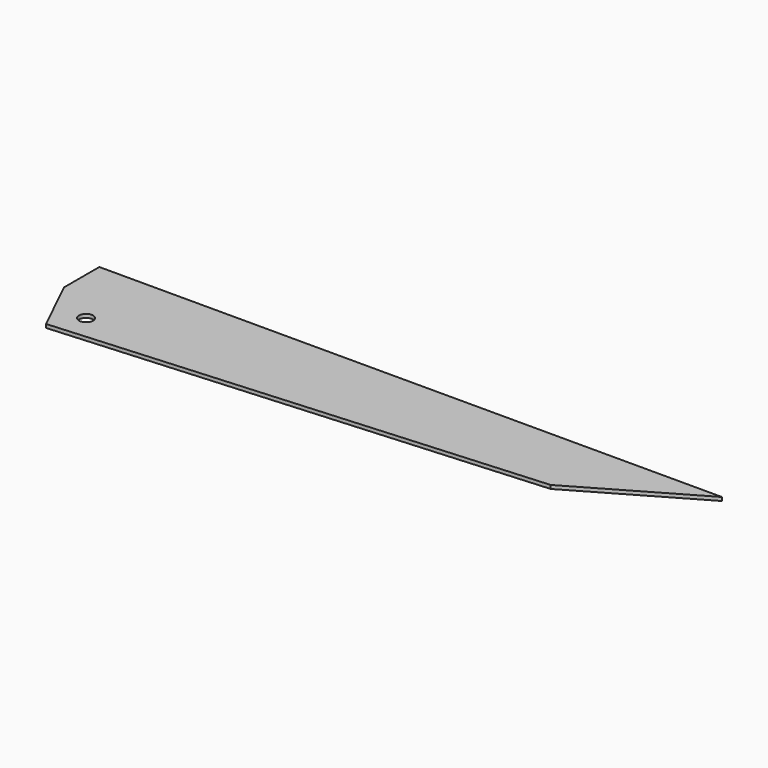
from build123d import *

# Parameters (mm, degrees)
F0_R     = 22.225
F0_R_2   = 6.35
F1_DEPTH = 3.175


# Not quite as in the source:
# - a feature names something its author has since deleted; it is built from what else it names


with BuildPart() as f1:
    # F0 (on Top) → F1 (new body)
    with BuildSketch(Plane.XY):
        Polygon((-217.8399659125, 274.6944633329), (-274.3403279131, 274.6944633329), (-249.4802269343, 223.6304721332), (-194.8479709943, 227.4676629604), align=None)
        with Locations((-233.2169740796, 248.1006040146)):
            Circle(F0_R, mode=Mode.SUBTRACT)
        with Locations((-233.2169740796, 248.1006040146)):
            Circle(F0_R)
        with Locations((-233.2169740796, 248.1006040146)):
            Circle(F0_R_2, mode=Mode.SUBTRACT)
        Polygon((-274.3403279131, 314.3819633329), (-274.3403279131, 274.6944633329), (-217.8399659125, 274.6944633329), (-233.0653279131, 305.9681798747), (-233.0653279131, 314.3819633329), align=None)
        Polygon((-233.0653279131, 305.9681798747), (-217.8399659125, 274.6944633329), (215.3278746861, 274.6944633329), (284.0686411115, 314.3819633329), (-233.0653279131, 314.3819633329), align=None)
        Polygon((215.3278746861, 274.6944633329), (-217.8399659125, 274.6944633329), (-194.8479709943, 227.4676629604), (179.0097919037, 253.726208462), align=None)
    extrude(amount=F1_DEPTH)


solid = f1.part
